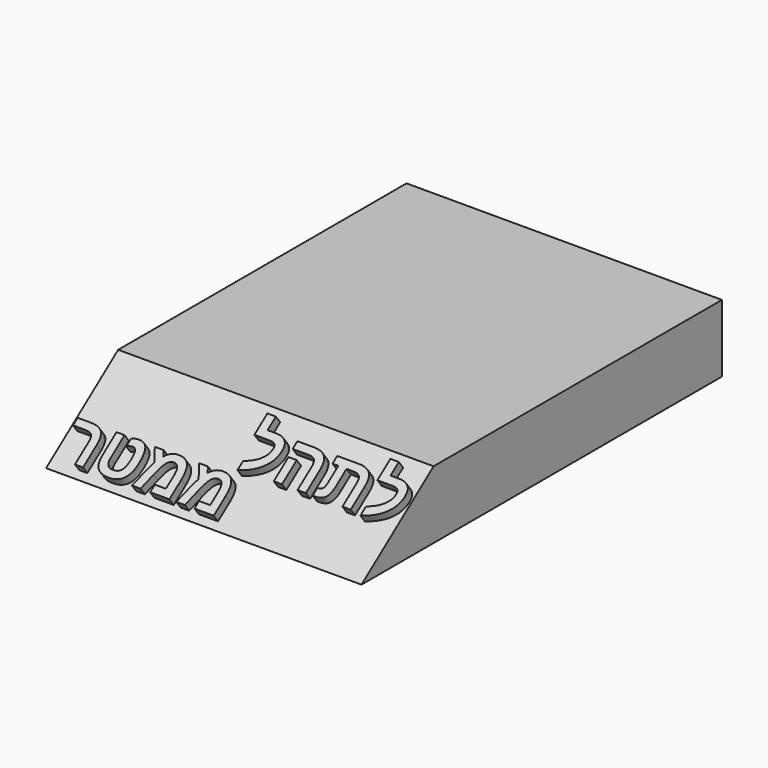
from build123d import *

# Parameters (mm, degrees)
F1_DEPTH       = 444.5
F2_TEXT_SIZE   = 176.3888888889
F2_TEXT_SIZE_2 = 172.0761289309
F3_DEPTH       = 25.4


# Not quite as in the source:
# - Text() gives the source's letters only with a copy of the font that has no kerning and outlines rounded to 1/6400 em; it was checked with that copy


with BuildPart() as f1:
    # F0 (on Right) → F1 (new body, symmetric)
    with BuildSketch(Plane.YZ):
        Polygon((-38.8390827179, -998.8214373589), (-38.8390827179, -808.3214373589), (-1054.8390827179, -808.3214373589), (-1308.8390827179, -998.8214373589), align=None)
    extrude(amount=F1_DEPTH, both=True)

    # F2 (on face) → F3 (join)
    with BuildSketch(Plane(origin=(0, 8.2522201538, -11.0029602051), x_dir=(1, 0, 0), z_dir=(0, -0.6, 0.8))):
        with Locations((0, -1499.9015035638)):
            Text('להתל', F2_TEXT_SIZE, font='Arimo', font_style=FontStyle.BOLD, text_align=(TextAlign.LEFT, TextAlign.BOTTOM))
        with Locations((-427.872911682, -1623.7963163941)):
            Text('רטממ', F2_TEXT_SIZE_2, font='Arimo', font_style=FontStyle.BOLD, text_align=(TextAlign.LEFT, TextAlign.BOTTOM))
    extrude(amount=F3_DEPTH)


solid = f1.part
